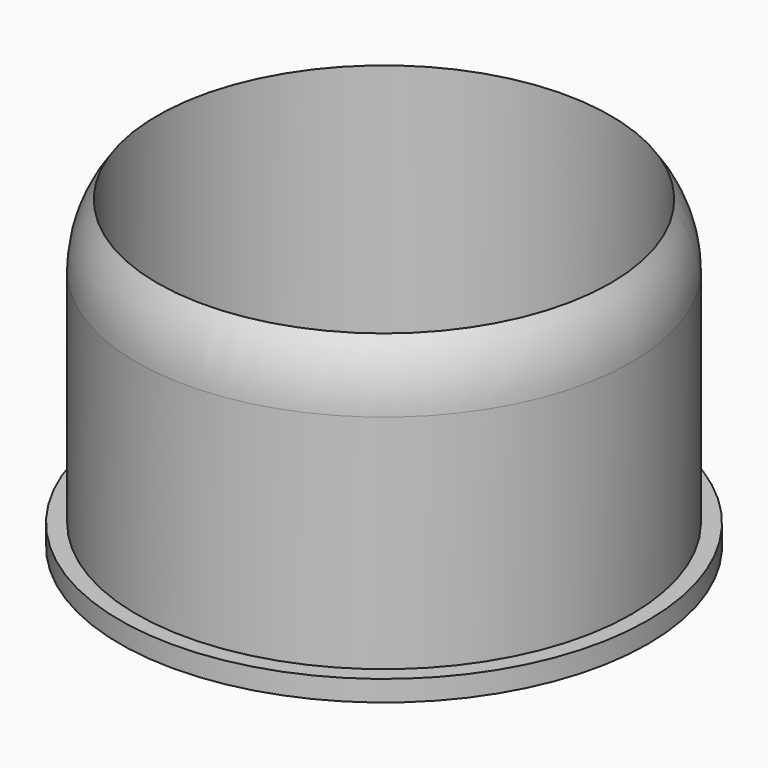
from build123d import *

# Parameters (mm, degrees)
F0_R     = 11.90625
F1_DEPTH = 12.7
F2_T     = -1
F3_DEPTH = 1
F4_R     = 12.7
F4_R_2   = 11.90625
F5_DEPTH = 1


# Not quite as in the source:
# - a fillet or chamfer that OpenCascade refuses, or shapes differently, is made with other operations: its cross-section is extruded or revolved along the edge and cut away or added


with BuildPart() as f1:
    # F0 (on Top) → F1 (new body)
    with BuildSketch(Plane.XY):
        Circle(F0_R)
    extrude(amount=F1_DEPTH)

    # F2
    f2_openings = [f1.faces().sort_by_distance(p)[0] for p in [
        (0, 0, 12.7),
    ]]
    offset(amount=F2_T, openings=f2_openings)

    # F3 (add): a face of the model
    f3_faces = [f1.faces().sort_by_distance(p)[0] for p in [
        (0, 0, 0),
    ]]
    extrude(f3_faces, amount=F3_DEPTH)

    # F6: fillet of radius 5.08 on 1 edges, made by hand

    # F6_s1 → F6_t2 (revolve, cut)
    with BuildSketch(Plane.XZ):
        with BuildLine():
            ThreePointArc((11.90625, 9.6734508099), (11.6497756815, 11.267188555), (10.90625, 12.7))
            Line((10.90625, 12.7), (11.90625, 12.7))
            Line((11.90625, 12.7), (11.90625, 9.6734508099))
        make_face()
    revolve(axis=Axis((0, 0, 12.7), (0, 0, 1)), mode=Mode.SUBTRACT)


with BuildPart() as f5:
    # F4 (on face) → F5 (new body)
    with BuildSketch(Plane(origin=(0, 0, -1), x_dir=(1, 0, 0), z_dir=(0, 0, -1))):
        Circle(F4_R)
        Circle(F4_R_2, mode=Mode.SUBTRACT)
        Circle(F4_R_2)
    extrude(amount=F5_DEPTH)


solid = Compound([f1.part, f5.part])
